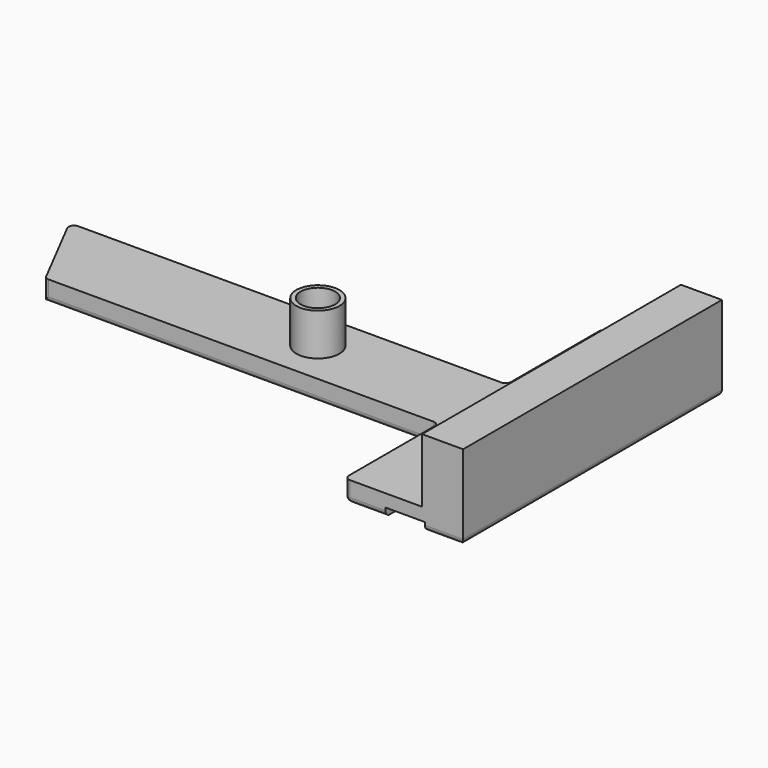
from build123d import *

# Parameters (mm, degrees)
F1_DEPTH = 0.9652
F2_W     = 1.905
F2_H     = 15.0368
F3_DEPTH = 2.9718
F2_R     = 1.0033
F2_R_2   = 0.8037883442
F4_DEPTH = 1.9558
F5_W     = 1.8288
F5_H     = 15.0368
F6_DEPTH = 0.381
F7_R     = 0.254


with BuildPart() as f1:
    # F0 (on Top) → F1 (new body)
    with BuildSketch(Plane.XY):
        Polygon((-2.7559, -7.5184), (2.7559, -7.5184), (2.7559, 7.5184), (0.8509, 7.5184), (-2.7559, 7.5184), (-2.7559, 1.905), (-23.0759, 1.905), (-21.0439, -2.035223273), (-2.7559, -2.035223273), align=None)
    extrude(amount=F1_DEPTH)

    # F2 (on face) → F3 (join)
    with BuildSketch(Plane.XY.offset(0.9652)):
        with Locations((1.8034, 0)):
            Rectangle(F2_W, F2_H)
    extrude(amount=F3_DEPTH)

    # F2 (on face) → F4 (join)
    with BuildSketch(Plane.XY.offset(0.9652)):
        with Locations((-10.0076, 0)):
            Circle(F2_R)
        with Locations((-10.0076, 0)):
            Circle(F2_R_2, mode=Mode.SUBTRACT)
    extrude(amount=F4_DEPTH)

    # F5 (on face) → F6 (cut)
    with BuildSketch(Plane(origin=(0, 0, 0), x_dir=(1, 0, 0), z_dir=(0, 0, -1))):
        with Locations((0.0654817199, 0)):
            Rectangle(F5_W, F5_H)
    extrude(amount=-F6_DEPTH, mode=Mode.SUBTRACT)

    # F7
    f7_edges = [f1.edges().sort_by_distance(p)[0] for p in [
        (-23.0759, 1.905, 0.4826),
        (-21.0439, -2.035223, 0.4826),
        (-2.7559, -7.5184, 0.4826),
        (-2.7559, 7.5184, 0.4826),
        (-2.7559, -2.035223, 0.4826),
        (-2.7559, 1.905, 0.4826),
        (-1.802409, 7.5184, 0),
        (1.867891, 7.5184, 0),
        (2.7559, 0, 0),
        (-2.7559, 4.7117, 0),
        (-2.7559, -4.776812, 0),
        (-1.802409, -7.5184, 0),
        (1.867891, -7.5184, 0),
        (-11.8999, -2.035223, 0),
        (-12.9159, 1.905, 0),
    ]]
    fillet(f7_edges, radius=F7_R)


solid = f1.part
